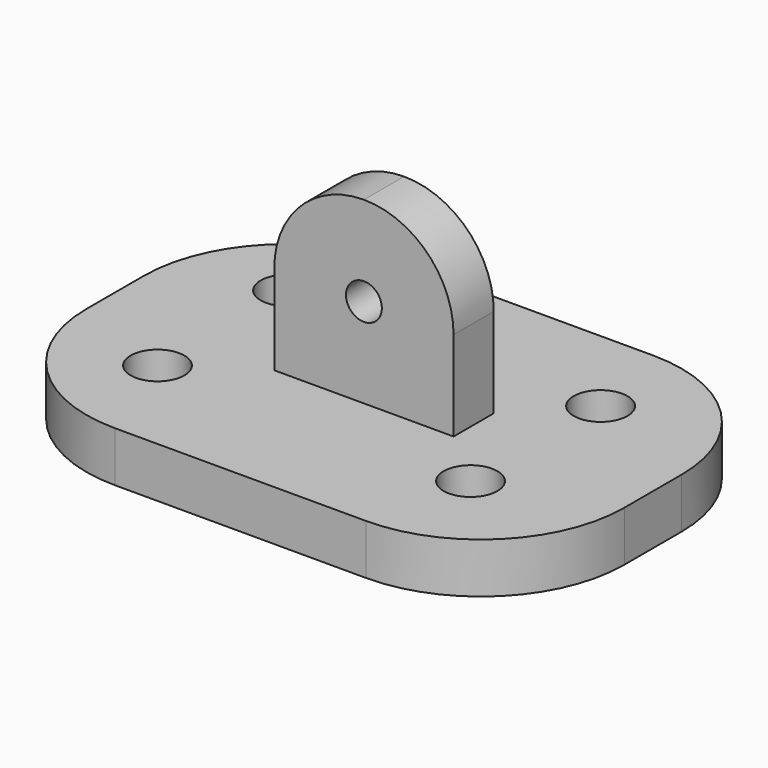
from build123d import *

# Parameters (mm, degrees)
F0_W     = 30
F0_H     = 20
F0_W_2   = 5
F0_H_2   = 2.8
F1_DEPTH = 2.8
F2_W     = 2.5
F2_H     = 2.8
F2_W_2   = 5
F3_DEPTH = 10
F5_D     = 2
F6_R     = 4.99999
F7_W     = 5
F7_H     = 2.8
F8_DEPTH = 2.8
F9_R     = 8
F11_D    = 3


# Not quite as in the source:
# - a fillet or chamfer is up to 0.001 mm smaller than in the source, because OpenCascade refuses the exact size


with BuildPart() as f1:
    # F0 (on Top) → F1 (new body)
    with BuildSketch(Plane.XY):
        with Locations((15, 10)):
            Rectangle(F0_W, F0_H)
        with Locations((15, 10)):
            Rectangle(F0_W_2, F0_H_2, mode=Mode.SUBTRACT)
    extrude(amount=F1_DEPTH)

    # F9
    f9_edges = [f1.edges().sort_by_distance(p)[0] for p in [
        (30, 20, 1.4),
        (0, 20, 1.4),
        (30, 0, 1.4),
        (0, 0, 1.4),
    ]]
    fillet(f9_edges, radius=F9_R)

    # F11 (through all)
    with Locations(Plane.XY.offset(2.8)):
        with Locations((5.7473420165, 14.8458313197), (23.2028886676, 14.8458313197), (23.2028886676, 5.7791140862), (5.7473420165, 5.7791140862)):
            Hole(F11_D / 2)


with BuildPart() as f3:
    # F2 (on face) → F3 (new body)
    with BuildSketch(Plane.XY.offset(2.8)):
        with Locations((18.75, 10)):
            Rectangle(F2_W, F2_H)
        with Locations((15, 10)):
            Rectangle(F2_W_2, F2_H)
        with Locations((11.25, 10)):
            Rectangle(F2_W, F2_H)
    extrude(amount=F3_DEPTH)

    # F5 (through all)
    with Locations(Plane.XZ.offset(-8.6)):
        with Locations((15, 7.8)):
            Hole(F5_D / 2)

    # F6 (radius 5 in the source; OpenCascade refuses exactly that, so slightly less here)
    f6_edges = [f3.edges().sort_by_distance(p)[0] for p in [
        (10, 10, 12.8),
        (20, 10, 12.8),
    ]]
    fillet(f6_edges, radius=F6_R)

    # F7 (on face) → F8 (join)
    with BuildSketch(Plane(origin=(0, 0, 2.8), x_dir=(1, 0, 0), z_dir=(0, 0, -1))):
        with Locations((15, -10)):
            Rectangle(F7_W, F7_H)
    extrude(amount=F8_DEPTH)


solid = Compound([f1.part, f3.part])
